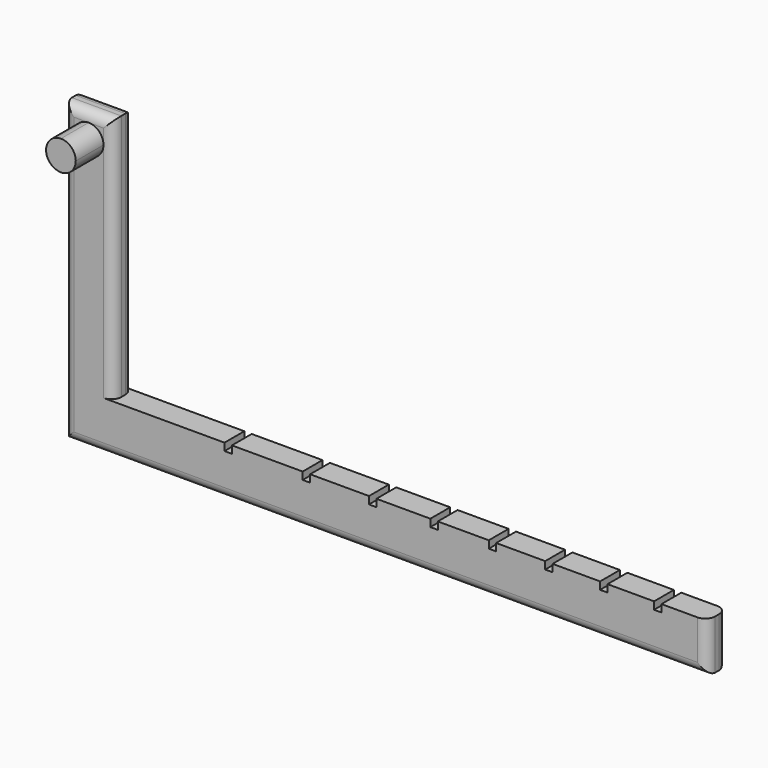
from build123d import *

# Parameters (mm, degrees)
F0_W     = 25.4
F0_H     = 127
F1_DEPTH = 12.7
F3_DEPTH = 17.78
F5_DEPTH = 25.4
F6_R     = 5.07999


# Not quite as in the source:
# - a fillet or chamfer is up to 0.001 mm smaller than in the source, because OpenCascade refuses the exact size


with BuildPart() as f1:
    # F0 (on Front) → F1 (new body)
    with BuildSketch(Plane.XZ):
        with Locations((12.7, 63.5)):
            Rectangle(F0_W, F0_H)
        Polygon((25.4, 0), (0, 0), (0, -25.4), (330.2, -25.4), (330.2, 0), align=None)
    extrude(amount=F1_DEPTH)

    # F2 (on face) → F3 (join)
    with BuildSketch(Plane.XZ.offset(12.7)):
        with BuildLine():
            ThreePointArc((12.7, 121.92), (7.3118463274, 108.9118463274), (20.32, 114.3))
            ThreePointArc((20.32, 114.3), (18.0881536726, 119.6881536726), (12.7, 121.92))
        make_face()
    extrude(amount=F3_DEPTH)

    # F4 (on face) → F5 (cut)
    with BuildSketch(Plane.XZ.offset(12.7)):
        Polygon((82.423, 3.81), (82.423, 0), (84.328, 0), (86.233, 0), (86.233, 3.81), align=None)
        Polygon((84.328, 0), (82.423, 0), (82.423, -3.81), (86.233, -3.81), (86.233, 0), align=None)
        Polygon((302.895, 3.81), (302.895, 0), (302.895, -3.81), (306.705, -3.81), (306.705, 3.81), align=None)
        Polygon((275.209, 3.81), (275.209, 0), (277.114, 0), (279.019, 0), (279.019, 3.81), align=None)
        Polygon((277.114, 0), (275.209, 0), (275.209, -3.81), (279.019, -3.81), (279.019, 0), align=None)
        Polygon((247.015, 3.81), (247.015, 0), (248.92, 0), (250.825, 0), (250.825, 3.81), align=None)
        Polygon((248.92, 0), (247.015, 0), (247.015, -3.81), (250.825, -3.81), (250.825, 0), align=None)
        Polygon((218.059, 3.81), (218.059, 0), (219.964, 0), (221.869, 0), (221.869, 3.81), align=None)
        Polygon((219.964, 0), (218.059, 0), (218.059, -3.81), (221.869, -3.81), (221.869, 0), align=None)
        Polygon((188.087, 3.81), (188.087, 0), (189.992, 0), (191.897, 0), (191.897, 3.81), align=None)
        Polygon((189.992, 0), (188.087, 0), (188.087, -3.81), (191.897, -3.81), (191.897, 0), align=None)
        Polygon((156.591, 3.81), (156.591, 0), (158.496, 0), (160.401, 0), (160.401, 3.81), align=None)
        Polygon((158.496, 0), (156.591, 0), (156.591, -3.81), (160.401, -3.81), (160.401, 0), align=None)
        Polygon((122.555, 3.81), (122.555, 0), (124.46, 0), (126.365, 0), (126.365, 3.81), align=None)
        Polygon((124.46, 0), (122.555, 0), (122.555, -3.81), (126.365, -3.81), (126.365, 0), align=None)
    extrude(amount=-F5_DEPTH, mode=Mode.SUBTRACT)

    # F6 (radius 5.08 in the source; OpenCascade refuses exactly that, so slightly less here)
    f6_edges = [f1.edges().sort_by_distance(p)[0] for p in [
        (165.1, -12.7, -25.4),
        (165.1, 0, -25.4),
        (0, 0, 50.8),
        (0, -12.7, 50.8),
        (12.7, 0, 127),
        (12.7, -12.7, 127),
        (25.4, 0, 63.5),
        (25.4, -12.7, 63.5),
        (330.2, 0, -12.7),
        (330.2, -12.7, -12.7),
    ]]
    fillet(f6_edges, radius=F6_R)


solid = f1.part
